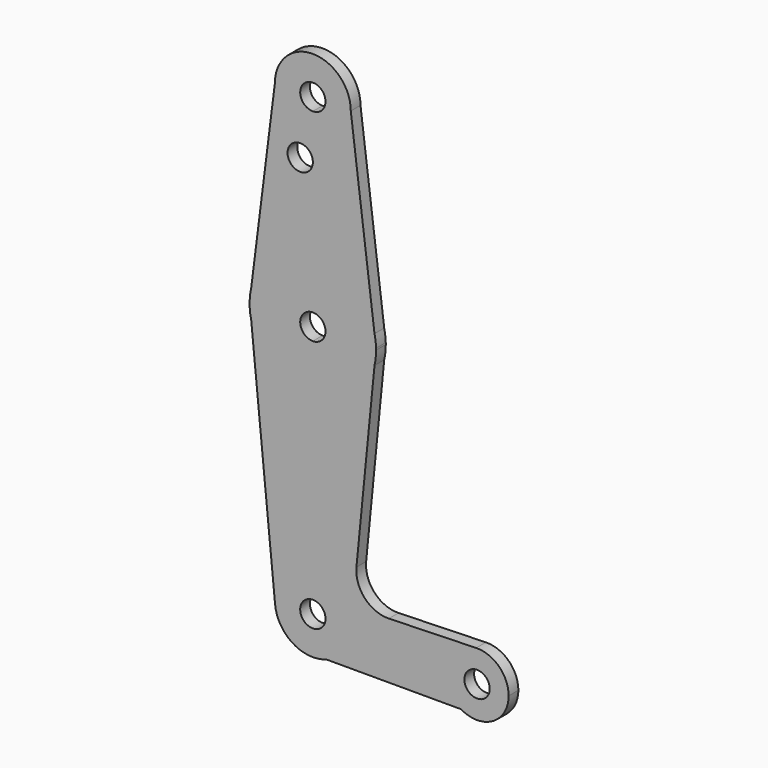
from build123d import *

# Parameters (mm, degrees)
F0_R     = 3.175
F1_DEPTH = 3.048


# Not quite as in the source:
# - a feature names something its author has since deleted; it is built from what else it names


with BuildPart() as f1:
    # F0 (on Front) → F1 (new body)
    with BuildSketch(Plane.XZ):
        with BuildLine():
            ThreePointArc((-25.2277835988, 89.1991540504), (-22.4379756896, 82.4639619596), (-15.7027835988, 79.6741540504))
            ThreePointArc((-15.7027835988, 79.6741540504), (-8.967591508, 82.4639619596), (-6.1777835988, 89.1991540504))
            ThreePointArc((-6.1777835988, 89.1991540504), (-15.7027835988, 98.7241540504), (-25.2277835988, 89.1991540504))
        make_face()
        with BuildLine():
            ThreePointArc((-12.5277835988, 89.1991540504), (-13.4577195686, 86.9540900201), (-15.7027835988, 86.0241540504))
            ThreePointArc((-15.7027835988, 86.0241540504), (-17.9478476291, 91.4442180807), (-12.5277835988, 89.1991540504))
        make_face(mode=Mode.SUBTRACT)
        with BuildLine():
            ThreePointArc((-6.1777835988, 89.1991540504), (-8.967591508, 82.4639619596), (-15.7027835988, 79.6741540504))
            Line((-15.7027835988, 79.6741540504), (-15.7027835988, 74.7860969014))
            Line((-15.7027835988, 74.7860969014), (-15.7027835988, 54.2741540504))
            ThreePointArc((-15.7027835988, 54.2741540504), (-5.7978377346, 50.8051071547), (-0.2218016911, 41.9140970332))
            Line((-0.2218016911, 41.9140970332), (-6.1777835988, 89.1991540504))
        make_face()
        with BuildLine():
            Line((-15.7027835988, 74.7860969014), (-15.7027835988, 79.6741540504))
            ThreePointArc((-15.7027835988, 79.6741540504), (-22.4379756896, 82.4639619596), (-25.2277835988, 89.1991540504))
            Line((-25.2277835988, 89.1991540504), (-31.1837655066, 41.9140970332))
            ThreePointArc((-31.1837655066, 41.9140970332), (-25.6077294631, 50.8051071547), (-15.7027835988, 54.2741540504))
            Line((-15.7027835988, 54.2741540504), (-15.7027835988, 74.7860969014))
        make_face()
        with Locations((-18.8777835988, 74.7860969014)):
            Circle(F0_R, mode=Mode.SUBTRACT)
        with BuildLine():
            ThreePointArc((-0.2218016911, 41.9140970332), (-5.7978377346, 50.8051071547), (-15.7027835988, 54.2741540504))
            Line((-15.7027835988, 54.2741540504), (-15.7027835988, 41.5741540504))
            ThreePointArc((-15.7027835988, 41.5741540504), (-13.4577195686, 40.6442180807), (-12.5277835988, 38.3991540504))
            ThreePointArc((-12.5277835988, 38.3991540504), (-13.4577195686, 36.1540900201), (-15.7027835988, 35.2241540504))
            Line((-15.7027835988, 35.2241540504), (-15.7027835988, 22.5241540504))
            ThreePointArc((-15.7027835988, 22.5241540504), (-5.8006414211, 25.990962994), (-0.2233918497, 34.8772148011))
            Line((-0.2233918497, 34.8772148011), (0.1662860895, 38.8330344781))
            Line((0.1662860895, 38.8330344781), (-0.2218016911, 41.9140970332))
        make_face()
        with BuildLine():
            Line((-15.7027835988, 41.5741540504), (-15.7027835988, 54.2741540504))
            ThreePointArc((-15.7027835988, 54.2741540504), (-25.6077294631, 50.8051071547), (-31.1837655066, 41.9140970332))
            Line((-31.1837655066, 41.9140970332), (-31.5718532872, 38.8330344781))
            Line((-31.5718532872, 38.8330344781), (-31.182175348, 34.8772148011))
            ThreePointArc((-31.182175348, 34.8772148011), (-25.6049257766, 25.990962994), (-15.7027835988, 22.5241540504))
            Line((-15.7027835988, 22.5241540504), (-15.7027835988, 35.2241540504))
            ThreePointArc((-15.7027835988, 35.2241540504), (-18.8777835988, 38.3991540504), (-15.7027835988, 41.5741540504))
        make_face()
        with BuildLine():
            Line((-31.5718532872, 38.8330344781), (-31.1837655066, 41.9140970332))
            ThreePointArc((-31.1837655066, 41.9140970332), (-31.4533286811, 40.3830780946), (-31.5718532872, 38.8330344781))
        make_face()
        with BuildLine():
            ThreePointArc((0.1662860895, 38.8330344781), (0.0477614834, 40.3830780946), (-0.2218016911, 41.9140970332))
            Line((-0.2218016911, 41.9140970332), (0.1662860895, 38.8330344781))
        make_face()
        with BuildLine():
            Line((-31.182175348, 34.8772148011), (-31.5718532872, 38.8330344781))
            ThreePointArc((-31.5718532872, 38.8330344781), (-31.5013163141, 36.8428799596), (-31.182175348, 34.8772148011))
        make_face()
        with BuildLine():
            ThreePointArc((0.1722164012, 38.3991540504), (0.170733754, 38.6161145273), (0.1662860895, 38.8330344781))
            Line((0.1662860895, 38.8330344781), (-0.2233918497, 34.8772148011))
            ThreePointArc((-0.2233918497, 34.8772148011), (0.0730043216, 36.6271098943), (0.1722164012, 38.3991540504))
        make_face()
        with BuildLine():
            ThreePointArc((-15.7027835988, 22.5241540504), (-25.6049257766, 25.990962994), (-31.182175348, 34.8772148011))
            Line((-31.182175348, 34.8772148011), (-25.181903228, -26.034610404))
            ThreePointArc((-25.181903228, -26.034610404), (-22.7603940807, -18.7043031892), (-15.7027835988, -15.5758459496))
            Line((-15.7027835988, -15.5758459496), (-15.7027835988, 22.5241540504))
        make_face()
        with BuildLine():
            Line((-4.7578265809, -11.1541468152), (-0.2233918497, 34.8772148011))
            ThreePointArc((-0.2233918497, 34.8772148011), (-5.8006414211, 25.990962994), (-15.7027835988, 22.5241540504))
            Line((-15.7027835988, 22.5241540504), (-15.7027835988, -15.5758459496))
            ThreePointArc((-15.7027835988, -15.5758459496), (-8.967591508, -18.3656538588), (-6.1777835988, -25.1008459496))
            ThreePointArc((-6.1777835988, -25.1008459496), (-7.8814722685, -30.5370867531), (-12.3830778926, -34.0286216538))
            Line((-12.3830778926, -34.0286216538), (21.5012593326, -34.0286216538))
            ThreePointArc((21.5012593326, -34.0286216538), (17.8308984551, -25.2118628548), (25.291047986, -19.2492330938))
            Line((25.291047986, -19.2492330938), (3.3830391656, -19.8804312387))
            ThreePointArc((3.3830391656, -19.8804312387), (-2.6591751738, -17.3567899438), (-4.7578265809, -11.1541468152))
        make_face()
        with BuildLine():
            ThreePointArc((-15.7027835988, -15.5758459496), (-22.7603940807, -18.7043031892), (-25.181903228, -26.034610404))
            ThreePointArc((-25.181903228, -26.034610404), (-23.2478837609, -30.9143722928), (-19.022489305, -34.0286216538))
            Line((-19.022489305, -34.0286216538), (-12.3830778926, -34.0286216538))
            ThreePointArc((-12.3830778926, -34.0286216538), (-7.8814722685, -30.5370867531), (-6.1777835988, -25.1008459496))
            ThreePointArc((-6.1777835988, -25.1008459496), (-8.967591508, -18.3656538588), (-15.7027835988, -15.5758459496))
        make_face()
        with BuildLine():
            ThreePointArc((-12.5277835988, -25.1008459496), (-17.9478476291, -27.3459099799), (-15.7027835988, -21.9258459496))
            ThreePointArc((-15.7027835988, -21.9258459496), (-13.4577195686, -22.8557819193), (-12.5277835988, -25.1008459496))
        make_face(mode=Mode.SUBTRACT)
        with BuildLine():
            Line((-12.3830778926, -34.0286216538), (-19.022489305, -34.0286216538))
            ThreePointArc((-19.022489305, -34.0286216538), (-15.7027835988, -34.6258459496), (-12.3830778926, -34.0286216538))
        make_face()
        with BuildLine():
            ThreePointArc((33.4571426277, -27.1834407253), (31.0508918664, -21.4905339011), (25.291047986, -19.2492330938))
            ThreePointArc((25.291047986, -19.2492330938), (17.8308984551, -25.2118628548), (21.5012593326, -34.0286216538))
            ThreePointArc((21.5012593326, -34.0286216538), (29.4634979017, -34.0718303649), (33.4571426277, -27.1834407253))
        make_face()
        with Locations((25.5196426277, -27.1834407253)):
            Circle(F0_R, mode=Mode.SUBTRACT)
    extrude(amount=F1_DEPTH)


solid = f1.part
